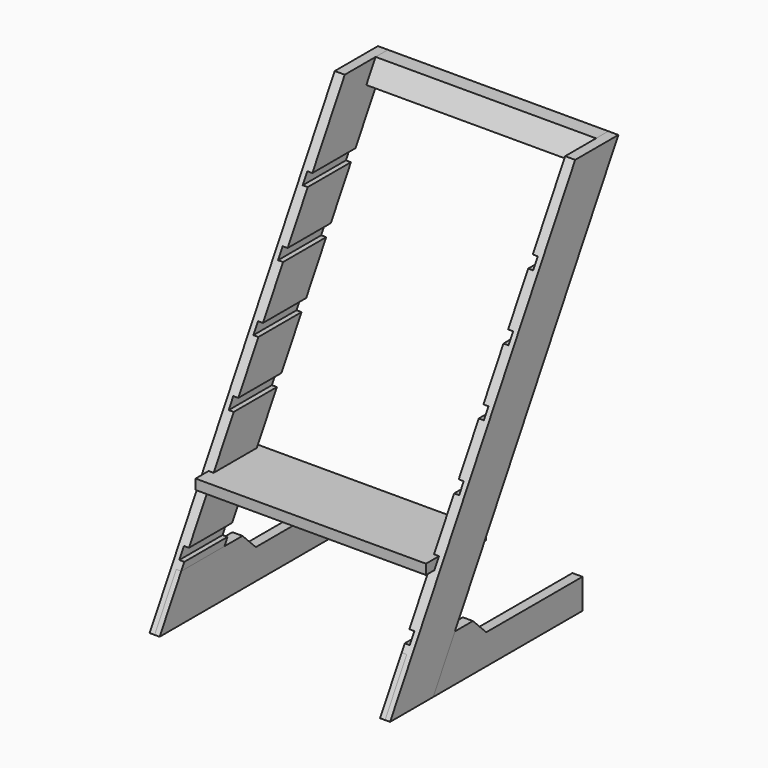
from build123d import *

# Parameters (mm, degrees)
F1_DEPTH  = 19.05
F3_DEPTH  = 9.525
F5_DEPTH  = 19.05
F7_DEPTH  = 9.525
F8_W      = 542.5937829844
F8_H      = 19.05
F9_DEPTH  = 9.525
F12_W     = 438.15
F12_H     = 142.875
F13_DEPTH = 19.05
F15_DEPTH = 419.1


# Not quite as in the source:
# - a length typed as a fraction of an inch, garbled in the dataset ("3 / 203.2 mm" for 3/8 in), is restored


with BuildPart() as f1:
    # F0 (on Right) → F1 (new body)
    with BuildSketch(Plane.YZ):
        Polygon((439.9409051225, 762), (0, 0), (102.6528778619, 0), (542.5937829844, 762), align=None)
    extrude(amount=F1_DEPTH)

    # F2 (on face) → F3 (cut)
    with BuildSketch(Plane.YZ.offset(19.05)):
        Polygon((51.326438931, 88.9), (0, 0), (102.6528778619, 0), (153.9793167929, 88.9), align=None)
    extrude(amount=-F3_DEPTH, mode=Mode.SUBTRACT)

    # F8 (on face) → F9 (cut)
    with BuildSketch(Plane.YZ.offset(19.05)):
        with Locations((271.2968914922, 111.125)):
            Rectangle(F8_W, F8_H)
        with Locations((271.2968914922, 212.725)):
            Rectangle(F8_W, F8_H)
        with Locations((271.2968914922, 314.325)):
            Rectangle(F8_W, F8_H)
        with Locations((271.2968914922, 415.925)):
            Rectangle(F8_W, F8_H)
        with Locations((271.2968914922, 517.525)):
            Rectangle(F8_W, F8_H)
        with Locations((271.2968914922, 619.125)):
            Rectangle(F8_W, F8_H)
    extrude(amount=-F9_DEPTH, mode=Mode.SUBTRACT)


with BuildPart() as f5:
    # F4 (on Right) → F5 (new body)
    with BuildSketch(Plane.YZ):
        Polygon((51.326438931, 88.9), (0, 0), (457.2, 0), (457.2, 57.15), (228.6, 57.15), (196.85, 88.9), align=None)
    extrude(amount=F5_DEPTH)

    # F6 (on face) → F7 (cut)
    with BuildSketch(Plane(origin=(0, 0, 0), x_dir=(0, -1, 0), z_dir=(-1, 0, 0))):
        Polygon((0, 0), (-51.326438931, 88.9), (-153.9793167929, 88.9), (-102.6528778619, 0), align=None)
    extrude(amount=-F7_DEPTH, mode=Mode.SUBTRACT)


with BuildPart() as f11_1:
    # F11: instance of F1
    add(f1.part.mirror(Plane.YZ.offset(228.6)))


with BuildPart() as f11_2:
    # F11: instance of F5
    add(f5.part.mirror(Plane.YZ.offset(228.6)))


with BuildPart() as f13:
    # F12 (on face) → F13 (new body)
    with BuildSketch(Plane.XY.offset(203.2)):
        with Locations((228.6, 168.6440136303)):
            Rectangle(F12_W, F12_H)
    extrude(amount=F13_DEPTH)


with BuildPart() as f15:
    # F14 (on face) → F15 (new body, through all)
    with BuildSketch(Plane.YZ.offset(19.05)):
        Polygon((520.5967377283, 723.9), (542.5937829844, 762), (513.2643893096, 762), (491.2673440535, 723.9), align=None)
    extrude(amount=F15_DEPTH)


solid = Compound([f1.part, f5.part, f11_1.part, f11_2.part, f13.part, f15.part])
